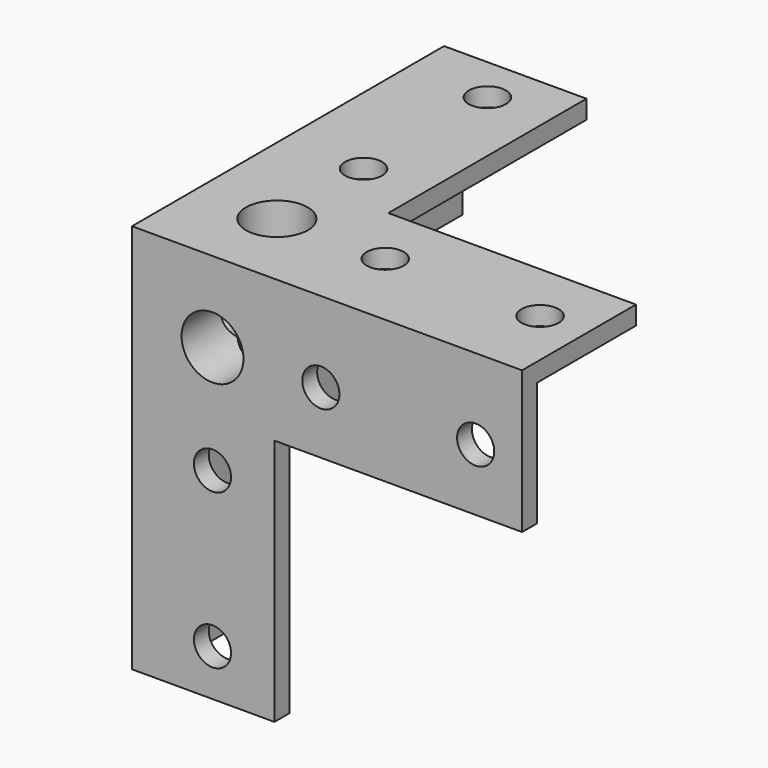
from build123d import *

# Parameters (mm, degrees)
F0_W                 = 20
F0_H                 = 40
F0_R                 = 3
F0_H_2               = 20
F0_R_2               = 5
F0_W_2               = 40
F1_DEPTH             = 3
F0_W_3               = 3
F0_H_3               = 3
F2_DEPTH             = 23
F3_DEPTH             = 63
F4_R                 = 3
F4_R_2               = 5
F6_DEPTH             = 25
F5_R                 = 3
F5_R_2               = 5
F7_DEPTH             = 25
F8_DEPTH             = 23
F9_D                 = 6
F9_DEPTH             = 23
F9_CBORE_D           = 10
F9_CBORE_DEPTH       = 21
F9_TIP               = 1.8025818571
F9_ON_F5_D           = 6
F9_ON_F5_DEPTH       = 23
F9_ON_F5_CBORE_D     = 10
F9_ON_F5_CBORE_DEPTH = 21
F9_ON_F5_TIP         = 1.8025818571
F9_ON_F4_D           = 6
F9_ON_F4_DEPTH       = 23
F9_ON_F4_CBORE_D     = 10
F9_ON_F4_CBORE_DEPTH = 21
F9_ON_F4_TIP         = 1.8025818571


# Not quite as in the source:
# - a feature of the source that left no trace in its solid (it failed there, or was rolled back) is left out


with BuildPart() as f1:
    # F0 (on Front) → F1 (new body)
    with BuildSketch(Plane.XZ):
        with Locations((-10, 20)):
            Rectangle(F0_W, F0_H)
        with Locations((-10, 7.5)):
            Circle(F0_R, mode=Mode.SUBTRACT)
        with Locations((-10, 32.5)):
            Circle(F0_R, mode=Mode.SUBTRACT)
        with Locations((-10, 50)):
            Rectangle(F0_W, F0_H_2)
        with Locations((-10, 50)):
            Circle(F0_R_2, mode=Mode.SUBTRACT)
        with Locations((20, 50)):
            Rectangle(F0_W_2, F0_H_2)
        with Locations((7.5, 50)):
            Circle(F0_R, mode=Mode.SUBTRACT)
        with Locations((32.5, 50)):
            Circle(F0_R, mode=Mode.SUBTRACT)
    extrude(amount=-F1_DEPTH)

    # F0 (on Front) → F2 (join)
    with BuildSketch(Plane.XZ):
        with Locations((-21.5, 20)):
            Rectangle(F0_W_3, F0_H)
        with Locations((20, 61.5)):
            Rectangle(F0_W_2, F0_H_3)
    extrude(amount=-F2_DEPTH)

    # F0 (on Front) → F3 (join)
    with BuildSketch(Plane.XZ):
        Polygon((-20, 60), (0, 60), (0, 63), (-23, 63), (-23, 60), align=None)
        with Locations((-21.5, 50)):
            Rectangle(F0_W_3, F0_H_2)
    extrude(amount=-F3_DEPTH)

    # F4 (on face) → F6 (cut)
    with BuildSketch(Plane.XY.offset(63)):
        with Locations((-10, 55.5)):
            Circle(F4_R)
        with Locations((-10, 30.5)):
            Circle(F4_R)
        with Locations((-10, 13)):
            Circle(F4_R_2)
        with Locations((7.5, 13)):
            Circle(F4_R)
        with Locations((32.5, 13)):
            Circle(F4_R)
    extrude(amount=-F6_DEPTH, mode=Mode.SUBTRACT)

    # F5 (on face) → F7 (cut)
    with BuildSketch(Plane(origin=(-23, 0, 0), x_dir=(0, -1, 0), z_dir=(-1, 0, 0))):
        with Locations((-55.5, 50)):
            Circle(F5_R)
        with Locations((-30.5, 50)):
            Circle(F5_R)
        with Locations((-13, 50)):
            Circle(F5_R_2)
        with Locations((-13, 7.5)):
            Circle(F5_R)
        with Locations((-13, 32.5)):
            Circle(F5_R)
    extrude(amount=-F7_DEPTH, mode=Mode.SUBTRACT)

    # F0 (on Front) → F8 (join)
    with BuildSketch(Plane.XZ):
        with Locations((-10, 50)):
            Rectangle(F0_W, F0_H_2)
        with Locations((-10, 50)):
            Circle(F0_R_2, mode=Mode.SUBTRACT)
        Polygon((-20, 60), (0, 60), (0, 63), (-23, 63), (-23, 60), align=None)
        with Locations((-21.5, 50)):
            Rectangle(F0_W_3, F0_H_2)
        with Locations((-10, 50)):
            Circle(F0_R_2)
    extrude(amount=-F8_DEPTH)

    # F9
    with Locations(Plane.XZ):
        with Locations((-10, 50)):
            CounterBoreHole(F9_D / 2, F9_CBORE_D / 2, F9_CBORE_DEPTH, depth=F9_DEPTH)
            with Locations((0, 0, -(F9_DEPTH + F9_TIP / 2))):  # 118° drill point
                Cone(0, F9_D / 2, F9_TIP, mode=Mode.SUBTRACT)

    # F9 on F5
    with Locations(Plane(origin=(-23, 0, 0), x_dir=(0, -1, 0), z_dir=(-1, 0, 0))):
        with Locations((-13, 50)):
            CounterBoreHole(F9_ON_F5_D / 2, F9_ON_F5_CBORE_D / 2, F9_ON_F5_CBORE_DEPTH, depth=F9_ON_F5_DEPTH)
            with Locations((0, 0, -(F9_ON_F5_DEPTH + F9_ON_F5_TIP / 2))):  # 118° drill point
                Cone(0, F9_ON_F5_D / 2, F9_ON_F5_TIP, mode=Mode.SUBTRACT)

    # F9 on F4
    with Locations(Plane.XY.offset(63)):
        with Locations((-10, 13)):
            CounterBoreHole(F9_ON_F4_D / 2, F9_ON_F4_CBORE_D / 2, F9_ON_F4_CBORE_DEPTH, depth=F9_ON_F4_DEPTH)
            with Locations((0, 0, -(F9_ON_F4_DEPTH + F9_ON_F4_TIP / 2))):  # 118° drill point
                Cone(0, F9_ON_F4_D / 2, F9_ON_F4_TIP, mode=Mode.SUBTRACT)


solid = f1.part
